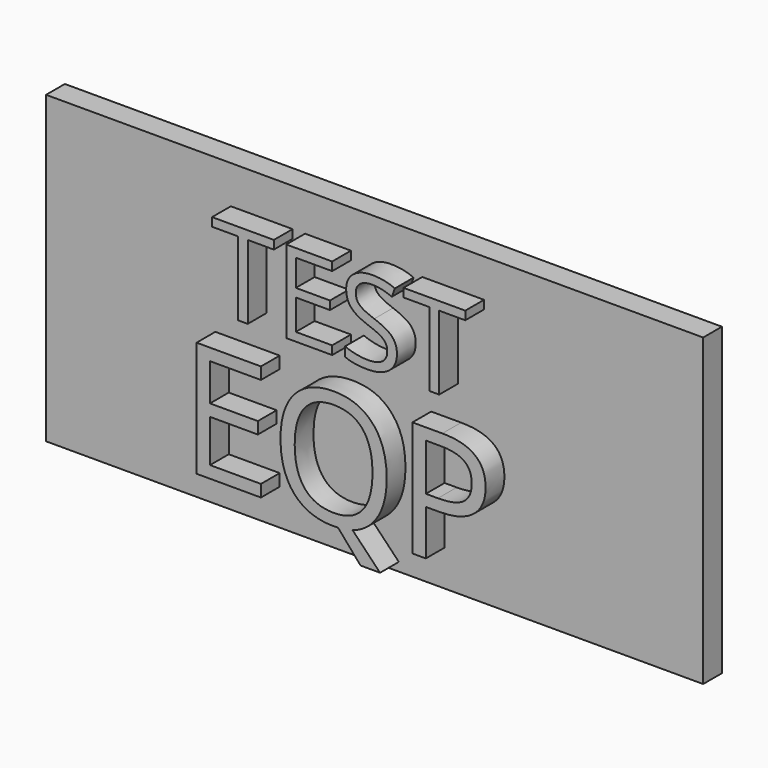
from build123d import *

# Parameters (mm, degrees)
F0_W           = 56
F0_H           = 26
F0_TEXT_SIZE   = 13.7795519549
F0_TEXT_SIZE_2 = 9.8377078151
F1_DEPTH       = 2
F2_DEPTH       = 2


# Not quite as in the source:
# - a feature names something its author has since deleted; it is built from what else it names
# - Text() gives the source's letters only with a copy of the font that has no kerning and outlines rounded to 1/6400 em; it was checked with that copy


with BuildPart() as f1:
    # F0 (on Front) → F1 (new body)
    with BuildSketch(Plane.XZ):
        with Locations((-28, 13)):
            Rectangle(F0_W, F0_H)
        Polygon((-36.0888848127, 4.0931811664), (-36.0888848127, 3.0704800447), (-41.5727158797, 3.0704800447), (-41.5727158797, 12.9077883075), (-36.0888848127, 12.9077883075), (-36.0888848127, 11.8915463509), (-40.4294436785, 11.8915463509), (-40.4294436785, 8.7222494012), (-36.3515575218, 8.7222494012), (-36.3515575218, 7.7124666095), (-40.4294436785, 7.7124666095), (-40.4294436785, 4.0931811664), align=None, mode=Mode.SUBTRACT)
        with BuildLine():
            add(Edge.make_bspline(
                [(-26.5616164688, 11.7171488964), (-25.3709770577, 10.3714895258), (-25.3709770577, 8.0031290336)],
                knots=[0, 0, 0, 1, 1, 1], degree=2))
            add(Edge.make_bspline(
                [(-25.3709770577, 8.0031290336), (-25.3709770577, 6.1127467497), (-26.1310054702, 4.8607452713)],
                knots=[0, 0, 0, 1, 1, 1], degree=2))
            add(Edge.make_bspline(
                [(-26.1310054702, 4.8607452713), (-26.8910338827, 3.6087437929), (-28.2776012982, 3.1652144644)],
                knots=[0, 0, 0, 1, 1, 1], degree=2))
            Line((-28.2776012982, 3.1652144644), (-25.9372305209, 0.7279562124))
            Line((-25.9372305209, 0.7279562124), (-27.5993889754, 0.7279562124))
            Line((-27.5993889754, 0.7279562124), (-29.5156079192, 2.9499089651))
            Line((-29.5156079192, 2.9499089651), (-29.885933378, 2.9348375801))
            add(Edge.make_bspline(
                [(-29.885933378, 2.9348375801), (-32.0583658659, 2.9348375801), (-33.2393165295, 4.2643490383)],
                knots=[0, 0, 0, 1, 1, 1], degree=2))
            add(Edge.make_bspline(
                [(-33.2393165295, 4.2643490383), (-34.4202671931, 5.5938604964), (-34.4202671931, 8.0160473635)],
                knots=[0, 0, 0, 1, 1, 1], degree=2))
            add(Edge.make_bspline(
                [(-34.4202671931, 8.0160473635), (-34.4202671931, 10.4188567357), (-33.236086947, 11.7408325013)],
                knots=[0, 0, 0, 1, 1, 1], degree=2))
            add(Edge.make_bspline(
                [(-33.236086947, 11.7408325013), (-32.0519067009, 13.062808267), (-29.873015048, 13.062808267)],
                knots=[0, 0, 0, 1, 1, 1], degree=2))
            add(Edge.make_bspline(
                [(-29.873015048, 13.062808267), (-27.7522558799, 13.062808267), (-26.5616164688, 11.7171488964)],
                knots=[0, 0, 0, 1, 1, 1], degree=2))
        make_face(mode=Mode.SUBTRACT)
        with BuildLine():
            add(Edge.make_bspline(
                [(-20.6277969082, 12.9077883075), (-16.9417667603, 12.9077883075), (-16.9417667603, 10.0420721119)],
                knots=[0, 0, 0, 1, 1, 1], degree=2))
            add(Edge.make_bspline(
                [(-16.9417667603, 10.0420721119), (-16.9417667603, 8.5478519468), (-17.9612382994, 7.7436859069)],
                knots=[0, 0, 0, 1, 1, 1], degree=2))
            add(Edge.make_bspline(
                [(-17.9612382994, 7.7436859069), (-18.9807098386, 6.939519867), (-20.8775512874, 6.939519867)],
                knots=[0, 0, 0, 1, 1, 1], degree=2))
            Line((-20.8775512874, 6.939519867), (-22.0358948736, 6.939519867))
            Line((-22.0358948736, 6.939519867), (-22.0358948736, 3.0704800447))
            Line((-22.0358948736, 3.0704800447), (-23.1791670749, 3.0704800447))
            Line((-23.1791670749, 3.0704800447), (-23.1791670749, 12.9077883075))
            Line((-23.1791670749, 12.9077883075), (-20.6277969082, 12.9077883075))
        make_face(mode=Mode.SUBTRACT)
        Polygon((-37.2120665779, 22.0318621274), (-37.2120665779, 15.7341919839), (-38.0282888982, 15.7341919839), (-38.0282888982, 22.0318621274), (-40.2525331495, 22.0318621274), (-40.2525331495, 22.7573930788), (-34.9878223266, 22.7573930788), (-34.9878223266, 22.0318621274), align=None, mode=Mode.SUBTRACT)
        Polygon((-30.0151684545, 16.4643343608), (-30.0151684545, 15.7341919839), (-33.9302687365, 15.7341919839), (-33.9302687365, 22.7573930788), (-30.0151684545, 22.7573930788), (-30.0151684545, 22.0318621274), (-33.1140464162, 22.0318621274), (-33.1140464162, 19.76918933), (-30.2026997597, 19.76918933), (-30.2026997597, 19.0482698041), (-33.1140464162, 19.0482698041), (-33.1140464162, 16.4643343608), align=None, mode=Mode.SUBTRACT)
        with BuildLine():
            add(Edge.make_bspline(
                [(-24.9118575254, 18.7746585555), (-24.4968292269, 18.3227388528), (-24.4968292269, 17.6033564688)],
                knots=[0, 0, 0, 1, 1, 1], degree=2))
            add(Edge.make_bspline(
                [(-24.4968292269, 17.6033564688), (-24.4968292269, 16.6764599356), (-25.1693287846, 16.1569059916)],
                knots=[0, 0, 0, 1, 1, 1], degree=2))
            add(Edge.make_bspline(
                [(-25.1693287846, 16.1569059916), (-25.8418283423, 15.6373520476), (-26.9946847269, 15.6373520476)],
                knots=[0, 0, 0, 1, 1, 1], degree=2))
            add(Edge.make_bspline(
                [(-26.9946847269, 15.6373520476), (-28.2428439059, 15.6373520476), (-28.9161120345, 15.9601518353)],
                knots=[0, 0, 0, 1, 1, 1], degree=2))
            Line((-28.9161120345, 15.9601518353), (-28.9161120345, 16.7471684605))
            add(Edge.make_bspline(
                [(-28.9161120345, 16.7471684605), (-28.4826380339, 16.5657857227), (-27.9738440828, 16.4597229353)],
                knots=[0, 0, 0, 1, 1, 1], degree=2))
            add(Edge.make_bspline(
                [(-27.9738440828, 16.4597229353), (-27.4650501318, 16.3536601479), (-26.9654790318, 16.3536601479)],
                knots=[0, 0, 0, 1, 1, 1], degree=2))
            add(Edge.make_bspline(
                [(-26.9654790318, 16.3536601479), (-26.1492567115, 16.3536601479), (-25.7357655549, 16.6633942299)],
                knots=[0, 0, 0, 1, 1, 1], degree=2))
            add(Edge.make_bspline(
                [(-25.7357655549, 16.6633942299), (-25.3222743983, 16.9731283119), (-25.3222743983, 17.5264993765)],
                knots=[0, 0, 0, 1, 1, 1], degree=2))
            add(Edge.make_bspline(
                [(-25.3222743983, 17.5264993765), (-25.3222743983, 17.890801994), (-25.4690714446, 18.1236789837)],
                knots=[0, 0, 0, 1, 1, 1], degree=2))
            add(Edge.make_bspline(
                [(-25.4690714446, 18.1236789837), (-25.6158684909, 18.3565559734), (-25.9594196935, 18.5540787006)],
                knots=[0, 0, 0, 1, 1, 1], degree=2))
            add(Edge.make_bspline(
                [(-25.9594196935, 18.5540787006), (-26.3029708961, 18.7516014278), (-27.0039075779, 19.0006184069)],
                knots=[0, 0, 0, 1, 1, 1], degree=2))
            add(Edge.make_bspline(
                [(-27.0039075779, 19.0006184069), (-27.9830669339, 19.3510867478), (-28.4034752288, 19.8314435747)],
                knots=[0, 0, 0, 1, 1, 1], degree=2))
            add(Edge.make_bspline(
                [(-28.4034752288, 19.8314435747), (-28.8238835237, 20.3118004016), (-28.8238835237, 21.0849827502)],
                knots=[0, 0, 0, 1, 1, 1], degree=2))
            add(Edge.make_bspline(
                [(-28.8238835237, 21.0849827502), (-28.8238835237, 21.896593645), (-28.2144067817, 22.3769504719)],
                knots=[0, 0, 0, 1, 1, 1], degree=2))
            add(Edge.make_bspline(
                [(-28.2144067817, 22.3769504719), (-27.6049300398, 22.8573072988), (-26.5996392724, 22.8573072988)],
                knots=[0, 0, 0, 1, 1, 1], degree=2))
            add(Edge.make_bspline(
                [(-26.5996392724, 22.8573072988), (-25.5528456752, 22.8573072988), (-24.6736005392, 22.4730218373)],
                knots=[0, 0, 0, 1, 1, 1], degree=2))
            Line((-24.6736005392, 22.4730218373), (-24.9287660857, 21.7628623044))
            add(Edge.make_bspline(
                [(-24.9287660857, 21.7628623044), (-25.7987883706, 22.1271649219), (-26.6196221164, 22.1271649219)],
                knots=[0, 0, 0, 1, 1, 1], degree=2))
            add(Edge.make_bspline(
                [(-26.6196221164, 22.1271649219), (-27.2682959755, 22.1271649219), (-27.6333671639, 21.8489422477)],
                knots=[0, 0, 0, 1, 1, 1], degree=2))
            add(Edge.make_bspline(
                [(-27.6333671639, 21.8489422477), (-27.9984383524, 21.5707195736), (-27.9984383524, 21.0757598992)],
                knots=[0, 0, 0, 1, 1, 1], degree=2))
            add(Edge.make_bspline(
                [(-27.9984383524, 21.0757598992), (-27.9984383524, 20.7114572816), (-27.8639384408, 20.477811721)],
                knots=[0, 0, 0, 1, 1, 1], degree=2))
            add(Edge.make_bspline(
                [(-27.8639384408, 20.477811721), (-27.7294385293, 20.2441661604), (-27.4097130253, 20.0497177169)],
                knots=[0, 0, 0, 1, 1, 1], degree=2))
            add(Edge.make_bspline(
                [(-27.4097130253, 20.0497177169), (-27.0899875213, 19.8552692733), (-26.4320908112, 19.6200865709)],
                knots=[0, 0, 0, 1, 1, 1], degree=2))
            add(Edge.make_bspline(
                [(-26.4320908112, 19.6200865709), (-25.3268858238, 19.2265782583), (-24.9118575254, 18.7746585555)],
                knots=[0, 0, 0, 1, 1, 1], degree=2))
        make_face(mode=Mode.SUBTRACT)
        Polygon((-20.8983801652, 22.0318621274), (-20.8983801652, 15.7341919839), (-21.7146024855, 15.7341919839), (-21.7146024855, 22.0318621274), (-23.9388467368, 22.0318621274), (-23.9388467368, 22.7573930788), (-18.6741359139, 22.7573930788), (-18.6741359139, 22.0318621274), align=None, mode=Mode.SUBTRACT)
        with BuildLine():
            add(Edge.make_bspline(
                [(-32.3587170374, 11.0066407487), (-33.2102502871, 9.9731743521), (-33.2102502871, 8.0031290336)],
                knots=[0, 0, 0, 1, 1, 1], degree=2))
            add(Edge.make_bspline(
                [(-33.2102502871, 8.0031290336), (-33.2102502871, 6.0050940001), (-32.3587170374, 4.9716276035)],
                knots=[0, 0, 0, 1, 1, 1], degree=2))
            add(Edge.make_bspline(
                [(-32.3587170374, 4.9716276035), (-31.5071837877, 3.9381612069), (-29.885933378, 3.9381612069)],
                knots=[0, 0, 0, 1, 1, 1], degree=2))
            add(Edge.make_bspline(
                [(-29.885933378, 3.9381612069), (-28.2517646383, 3.9381612069), (-27.4174558285, 4.9673214935)],
                knots=[0, 0, 0, 1, 1, 1], degree=2))
            add(Edge.make_bspline(
                [(-27.4174558285, 4.9673214935), (-26.5831470188, 5.9964817801), (-26.5831470188, 8.0031290336)],
                knots=[0, 0, 0, 1, 1, 1], degree=2))
            add(Edge.make_bspline(
                [(-26.5831470188, 8.0031290336), (-26.5831470188, 9.9882457371), (-27.414226246, 11.0141764412)],
                knots=[0, 0, 0, 1, 1, 1], degree=2))
            add(Edge.make_bspline(
                [(-27.414226246, 11.0141764412), (-28.2453054733, 12.0401071454), (-29.873015048, 12.0401071454)],
                knots=[0, 0, 0, 1, 1, 1], degree=2))
            add(Edge.make_bspline(
                [(-29.873015048, 12.0401071454), (-31.5071837877, 12.0401071454), (-32.3587170374, 11.0066407487)],
                knots=[0, 0, 0, 1, 1, 1], degree=2))
        make_face()
        with Locations((-42.9248344153, 3.0704800447)):
            Text('EQP', F0_TEXT_SIZE, font='Open Sans', text_align=(TextAlign.LEFT, TextAlign.BOTTOM))
        with BuildLine():
            Line((-22.0358948736, 11.9173830108), (-22.0358948736, 7.9213129438))
            Line((-22.0358948736, 7.9213129438), (-21.004581532, 7.9213129438))
            add(Edge.make_bspline(
                [(-21.004581532, 7.9213129438), (-19.484524707, 7.9213129438), (-18.8052358567, 8.4122094822)],
                knots=[0, 0, 0, 1, 1, 1], degree=2))
            add(Edge.make_bspline(
                [(-18.8052358567, 8.4122094822), (-18.1259470064, 8.9031060206), (-18.1259470064, 9.9882457371)],
                knots=[0, 0, 0, 1, 1, 1], degree=2))
            add(Edge.make_bspline(
                [(-18.1259470064, 9.9882457371), (-18.1259470064, 10.9635796489), (-18.7654043393, 11.4404813298)],
                knots=[0, 0, 0, 1, 1, 1], degree=2))
            add(Edge.make_bspline(
                [(-18.7654043393, 11.4404813298), (-19.4048616722, 11.9173830108), (-20.7569802078, 11.9173830108)],
                knots=[0, 0, 0, 1, 1, 1], degree=2))
            Line((-20.7569802078, 11.9173830108), (-22.0358948736, 11.9173830108))
        make_face()
        with Locations((-40.3386130929, 15.7341919839)):
            Text('TEST', F0_TEXT_SIZE_2, font='Open Sans', text_align=(TextAlign.LEFT, TextAlign.BOTTOM))
    extrude(amount=-F1_DEPTH)

    # F0 (on Front) → F2 (join)
    with BuildSketch(Plane.XZ):
        with Locations((-42.9248344153, 3.0704800447)):
            Text('EQP', F0_TEXT_SIZE, font='Open Sans', text_align=(TextAlign.LEFT, TextAlign.BOTTOM))
        with Locations((-40.3386130929, 15.7341919839)):
            Text('TEST', F0_TEXT_SIZE_2, font='Open Sans', text_align=(TextAlign.LEFT, TextAlign.BOTTOM))
    extrude(amount=F2_DEPTH)


solid = f1.part
